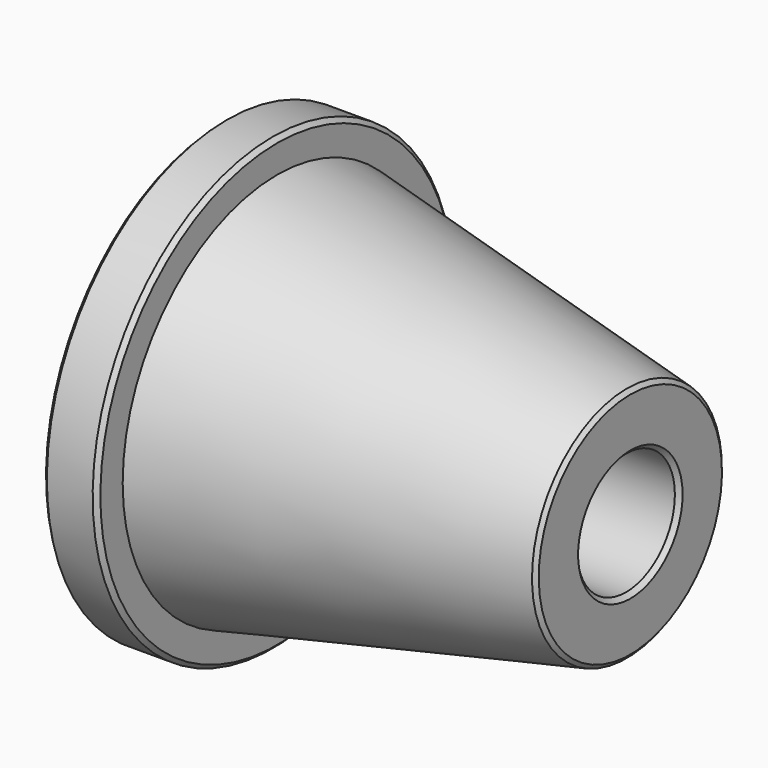
from build123d import *

# Parameters (mm, degrees)
F3_D = 36.11626


# Not quite as in the source:
# - a fillet or chamfer that OpenCascade refuses, or shapes differently, is made with other operations: its cross-section is extruded or revolved along the edge and cut away or added


with BuildPart() as f1:
    # F0 (on Front) → F1 (revolve)
    with BuildSketch(Plane.XZ):
        Polygon((0, 0), (0, 34.925), (-104.5604041832, 57.15), (-104.5604041832, 66.675), (-120.65, 66.675), (-120.65, 20.32), (-55.88, 20.32), (-55.88, 0), align=None)
    revolve(axis=Axis((-55.6578852736, 0, 0), (-1, 0, 0)))

    # F3 (through all)
    with Locations(Plane.YZ):
        with Locations((0, 0)):
            Hole(F3_D / 2)

    # F4: chamfer of 1.27 on 5 edges, made by hand

    # F4_s1 → F4_t2 (revolve, cut)
    with BuildSketch(Plane.XZ):
        Polygon((-120.65, 65.405), (-119.38, 66.675), (-120.65, 66.675), align=None)
    revolve(axis=Axis((-120.65, 0, 0), (-1, 0, 0)), mode=Mode.SUBTRACT)

    # F4_s3 → F4_t4 (revolve, cut)
    with BuildSketch(Plane.XZ):
        Polygon((-119.38, 20.32), (-120.65, 21.59), (-120.65, 20.32), align=None)
    revolve(axis=Axis((-120.65, 0, 0), (-1, 0, 0)), mode=Mode.SUBTRACT)

    # F4_s5 → F4_t6 (revolve, cut)
    with BuildSketch(Plane.XZ):
        Polygon((-105.8304041832, 66.675), (-104.5604041832, 65.405), (-104.5604041832, 66.675), align=None)
    revolve(axis=Axis((-104.5604041832, 0, 0), (-1, 0, 0)), mode=Mode.SUBTRACT)

    # F4_s7 → F4_t8 (revolve, cut)
    with BuildSketch(Plane.XZ):
        Polygon((0, 33.8965742778), (-1.0059521527, 35.1388217308), (0, 34.925), align=None)
    revolve(axis=Axis((0, 0, 0), (-1, 0, 0)), mode=Mode.SUBTRACT)

    # F4_s9 → F4_t10 (revolve, cut)
    with BuildSketch(Plane.XY):
        Polygon((-1.27, 18.05813), (0, 19.32813), (0, 18.05813), align=None)
    revolve(axis=Axis((0, 0, 0), (1, 0, 0)), mode=Mode.SUBTRACT)


solid = f1.part
